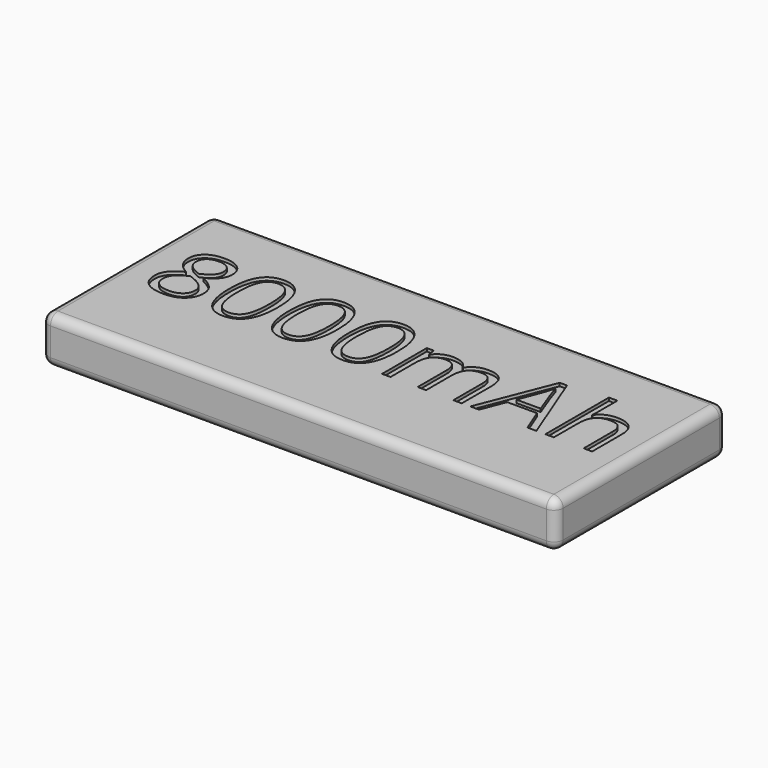
from build123d import *

# Parameters (mm, degrees)
F0_W         = 166
F0_H         = 69
F1_DEPTH     = 15
F2_R         = 3
F3_TEXT_SIZE = 33.7232585099
F4_DEPTH     = 1


# Not quite as in the source:
# - Text() gives the source's letters only with a copy of the font that has no kerning and outlines rounded to 1/6400 em; it was checked with that copy


with BuildPart() as f1:
    # F0 (on Top) → F1 (new body)
    with BuildSketch(Plane.XY):
        Rectangle(F0_W, F0_H)
    extrude(amount=F1_DEPTH)

    # F2
    f2_edges = [f1.edges().sort_by_distance(p)[0] for p in [
        (0, -34.5, 15),
        (83, 0, 15),
        (0, 34.5, 15),
        (-83, 0, 15),
        (0, -34.5, 0),
        (83, 0, 0),
        (0, 34.5, 0),
        (-83, 0, 0),
        (-83, -34.5, 7.5),
        (-83, 34.5, 7.5),
        (83, -34.5, 7.5),
        (83, 34.5, 7.5),
    ]]
    fillet(f2_edges, radius=F2_R)

    # F3 (on face) → F4 (cut)
    with BuildSketch(Plane.XY.offset(15)):
        with Locations((-74.8622540526, -7.2375191293)):
            Text('8000mAh', F3_TEXT_SIZE, font='Open Sans', text_align=(TextAlign.LEFT, TextAlign.BOTTOM))
    extrude(amount=-F4_DEPTH, mode=Mode.SUBTRACT)


solid = f1.part
